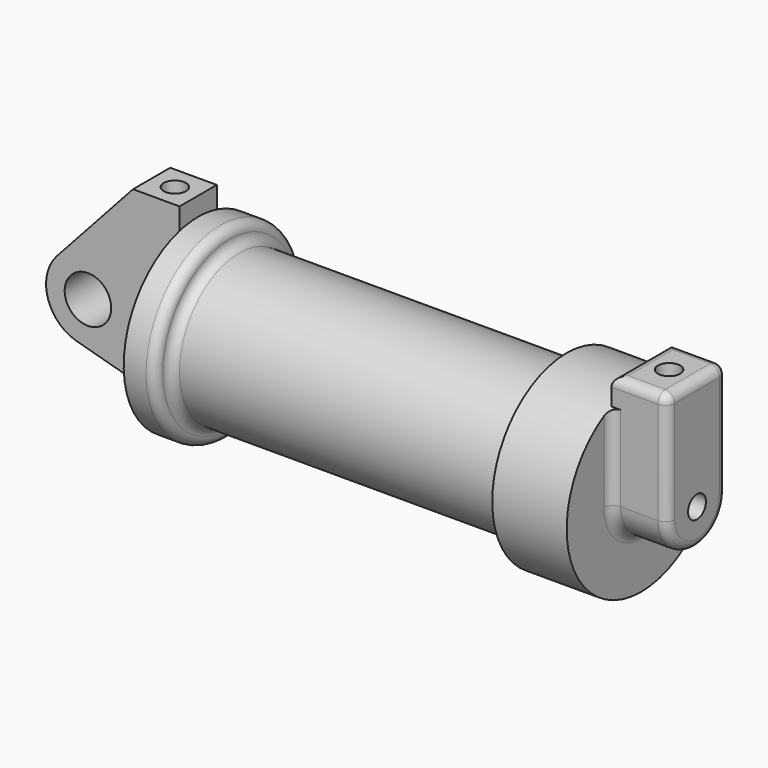
from build123d import *

# Parameters (mm, degrees)
F0_W          = 5.842
F0_H          = 12.7
F0_R          = 3.175
F2_DEPTH      = 3.175
F3_R          = 1.524
F4_DEPTH      = 7.62
F5_R          = 1.524
F7_DEPTH      = 17.78
F6_R          = 1.524
F8_DEPTH      = 10.414
F9_R          = 1.26999
F10_T4_DEPTH  = 14.8147422652
F10_S5_R      = 12.7
F10_T6_DEPTH  = 9
F10_T10_DEPTH = 14.8147422652
F10_S11_R     = 12.7
F10_T12_DEPTH = 9
F10_T14_ANGLE = 180
F10_T15_DEPTH = 13.97
F10_T17_DEPTH = 7.62
F10_T19_DEPTH = 16.51
F10_T21_DEPTH = 9.525
F10_S25_W     = 1.2954
F10_S25_H     = 1.2954
F10_T26_DEPTH = 1.2954
F10_S31_W     = 1.2954
F10_S31_H     = 1.2954
F10_T32_DEPTH = 1.2954
F10_T36_ANGLE = 180


# Not quite as in the source:
# - a fillet or chamfer that OpenCascade refuses, or shapes differently, is made with other operations: its cross-section is extruded or revolved along the edge and cut away or added
# - a fillet or chamfer is up to 0.001 mm smaller than in the source, because OpenCascade refuses the exact size


with BuildPart() as f1:
    # F0 (on Front) → F1 (revolve)
    with BuildSketch(Plane.XZ):
        Polygon((5.842, 12.7), (5.842, 0), (66.294, 0), (66.294, 12.7), (56.134, 12.7), (56.134, 10.16), (10.16, 10.16), (10.16, 12.7), align=None)
    revolve(axis=Axis((33.147, 0, 0), (-1, 0, 0)))

    # F0 (on Front) → F2 (join, symmetric)
    with BuildSketch(Plane.XZ):
        with BuildLine():
            Line((5.842, 0), (0, 0))
            Line((0, 0), (-0.9398, 0))
            ThreePointArc((-0.9398, 0), (-3.1957909266, -4.5493385486), (-8.1826630726, -5.5069827884))
            Line((-8.1826630726, -5.5069827884), (5.842, -9.398))
            Line((5.842, -9.398), (5.842, 0))
        make_face()
        with BuildLine():
            Line((-0.9398, 0), (0, 0))
            Line((0, 0), (0, 12.7))
            Line((0, 12.7), (5.842, 12.7))
            Line((5.842, 12.7), (5.842, 15.24))
            Line((5.842, 15.24), (-0.508, 15.24))
            Line((-0.508, 15.24), (-10.8806298187, 3.8475430269))
            ThreePointArc((-10.8806298187, 3.8475430269), (-4.5919612295, 5.3297205562), (-0.9398, 0))
        make_face()
        with Locations((2.921, 6.35)):
            Rectangle(F0_W, F0_H)
        with BuildLine():
            ThreePointArc((-8.1826630726, -5.5069827884), (-3.1957909266, -4.5493385486), (-0.9398, 0))
            ThreePointArc((-0.9398, 0), (-4.5919612295, 5.3297205562), (-10.8806298187, 3.8475430269))
            ThreePointArc((-10.8806298187, 3.8475430269), (-12.1459778134, -1.5837270034), (-8.1826630726, -5.5069827884))
        make_face()
        with Locations((-6.6548, 0)):
            Circle(F0_R, mode=Mode.SUBTRACT)
    extrude(amount=F2_DEPTH, both=True)

    # F3 (on face) → F4 (join)
    with BuildSketch(Plane.YZ.offset(66.294)):
        with BuildLine():
            ThreePointArc((-5.08, 0), (0, -5.08), (5.08, 0))
            ThreePointArc((5.08, 0), (0, 5.08), (-5.08, 0))
        make_face()
        Circle(F3_R, mode=Mode.SUBTRACT)
        with BuildLine():
            ThreePointArc((-5.08, 0), (0, 5.08), (5.08, 0))
            Line((5.08, 0), (5.08, 15.24))
            Line((5.08, 15.24), (-5.08, 15.24))
            Line((-5.08, 15.24), (-5.08, 0))
        make_face()
    extrude(amount=F4_DEPTH)

    # F5 (on face) → F7 (cut)
    with BuildSketch(Plane.XY.offset(15.24)):
        with Locations((2.667, 0)):
            Circle(F5_R)
    extrude(amount=-F7_DEPTH, mode=Mode.SUBTRACT)

    # F6 (on face) → F8 (cut)
    with BuildSketch(Plane.XY.offset(15.24)):
        with Locations((70.104, 0)):
            Circle(F6_R)
    extrude(amount=-F8_DEPTH, mode=Mode.SUBTRACT)

    # F9 (radius 1.27 in the source; OpenCascade refuses exactly that, so slightly less here)
    f9_edges = [f1.edges().sort_by_distance(p)[0] for p in [
        (10.16, 0, -12.7),
        (10.16, 0, -10.16),
    ]]
    fillet(f9_edges, radius=F9_R)

    # F10: fillet of radius 1.27 on 12 edges, made by hand


with BuildPart() as f10_tool2:
    # F10_s3 → F10_t4 (new body)
    with BuildSketch(Plane.XY.offset(14.8147422652)):
        with BuildLine():
            ThreePointArc((66.294, -6.35), (66.6659743879, -5.4519743879), (67.564, -5.08))
            Line((67.564, -5.08), (66.294, -5.08))
            Line((66.294, -5.08), (66.294, -6.35))
        make_face()
    extrude(amount=-F10_T4_DEPTH)

    # F10_s5 → F10_t6 (intersect, symmetric)
    with BuildSketch(Plane.YZ.offset(66.9)):
        Circle(F10_S5_R)
    extrude(amount=F10_T6_DEPTH, both=True, mode=Mode.INTERSECT)


with BuildPart() as f1_1:
    add(f1.part)

    # F10_t1: union F10_tool2
    add(f10_tool2.part)


with BuildPart() as f10_tool8:
    # F10_s9 → F10_t10 (new body)
    with BuildSketch(Plane.XY):
        with BuildLine():
            ThreePointArc((66.294, 6.35), (66.6659743879, 5.4519743879), (67.564, 5.08))
            Line((67.564, 5.08), (66.294, 5.08))
            Line((66.294, 5.08), (66.294, 6.35))
        make_face()
    extrude(amount=F10_T10_DEPTH)

    # F10_s11 → F10_t12 (intersect, symmetric)
    with BuildSketch(Plane.YZ.offset(66.9)):
        Circle(F10_S11_R)
    extrude(amount=F10_T12_DEPTH, both=True, mode=Mode.INTERSECT)


with BuildPart() as f1_2:
    add(f1_1.part)

    # F10_t7: union F10_tool8
    add(f10_tool8.part)

    # F10_s13 → F10_t14 (revolve)
    with BuildSketch(Plane.XY):
        with BuildLine():
            ThreePointArc((66.294, -6.35), (66.6659743879, -5.4519743879), (67.564, -5.08))
            Line((67.564, -5.08), (66.294, -5.08))
            Line((66.294, -5.08), (66.294, -6.35))
        make_face()
    revolve(axis=Axis((66.294, 0, 0), (1, 0, 0)), revolution_arc=F10_T14_ANGLE)

    # F10_s16 → F10_t15 (cut)
    with BuildSketch(Plane.XY):
        with BuildLine():
            ThreePointArc((72.644, 5.08), (73.5420256121, 4.7080256121), (73.914, 3.81))
            Line((73.914, 3.81), (73.914, 5.08))
            Line((73.914, 5.08), (72.644, 5.08))
        make_face()
        with BuildLine():
            ThreePointArc((72.644, -5.08), (73.5420256121, -4.7080256121), (73.914, -3.81))
            Line((73.914, -3.81), (73.914, -5.08))
            Line((73.914, -5.08), (72.644, -5.08))
        make_face()
    extrude(amount=F10_T15_DEPTH, mode=Mode.SUBTRACT)

    # F10_s18 → F10_t17 (cut)
    with BuildSketch(Plane.XZ.offset(-3.81)):
        with BuildLine():
            ThreePointArc((72.644, 15.24), (73.5420256121, 14.8680256121), (73.914, 13.97))
            Line((73.914, 13.97), (73.914, 15.24))
            Line((73.914, 15.24), (72.644, 15.24))
        make_face()
    extrude(amount=F10_T17_DEPTH, mode=Mode.SUBTRACT)

    # F10_s20 → F10_t19 (cut)
    with BuildSketch(Plane.XZ.offset(-8.255)):
        with BuildLine():
            ThreePointArc((66.294, 13.97), (66.6659743879, 14.8680256121), (67.564, 15.24))
            Line((67.564, 15.24), (66.294, 15.24))
            Line((66.294, 15.24), (66.294, 13.97))
        make_face()
    extrude(amount=F10_T19_DEPTH, mode=Mode.SUBTRACT)

    # F10_s22 → F10_t21 (cut)
    with BuildSketch(Plane.YZ.offset(63.119)):
        with BuildLine():
            ThreePointArc((3.81, 15.24), (4.7080256121, 14.8680256121), (5.08, 13.97))
            Line((5.08, 13.97), (5.08, 15.24))
            Line((5.08, 15.24), (3.81, 15.24))
        make_face()
        with BuildLine():
            ThreePointArc((-5.08, 13.97), (-4.7080256121, 14.8680256121), (-3.81, 15.24))
            Line((-3.81, 15.24), (-5.08, 15.24))
            Line((-5.08, 15.24), (-5.08, 13.97))
        make_face()
    extrude(amount=F10_T21_DEPTH, mode=Mode.SUBTRACT)


with BuildPart() as f10_tool24:
    # F10_s25 → F10_t26 (new body)
    with BuildSketch(Plane.XY.offset(13.97)):
        with Locations((73.2917, 4.4577)):
            Rectangle(F10_S25_W, F10_S25_H)
    extrude(amount=F10_T26_DEPTH)

    # F10_s27 → F10_t28 (revolve, cut)
    with BuildSketch(Plane(origin=(72.644, 3.81, 13.97), x_dir=(-0.7071067812, -0.7071067812, 0), z_dir=(-0.7071067812, 0.7071067812, 0))):
        with BuildLine():
            ThreePointArc((0, -1.27), (1.27, 0), (0, 1.27))
            Line((0, 1.27), (0, -1.27))
        make_face()
    revolve(axis=Axis((72.644, 3.81, 13.97), (0, 0, 1)), mode=Mode.SUBTRACT)


with BuildPart() as f1_3:
    add(f1_2.part)

    # F10_t23: cut F10_tool24
    add(f10_tool24.part, mode=Mode.SUBTRACT)


with BuildPart() as f10_tool30:
    # F10_s31 → F10_t32 (new body)
    with BuildSketch(Plane.XZ.offset(3.81)):
        with Locations((73.2917, 14.6177)):
            Rectangle(F10_S31_W, F10_S31_H)
    extrude(amount=F10_T32_DEPTH)

    # F10_s33 → F10_t34 (revolve, cut)
    with BuildSketch(Plane(origin=(72.644, -3.81, 13.97), x_dir=(-0.7071067812, 0, -0.7071067812), z_dir=(-0.7071067812, 0, 0.7071067812))):
        with BuildLine():
            ThreePointArc((0, -1.27), (1.27, 0), (0, 1.27))
            Line((0, 1.27), (0, -1.27))
        make_face()
    revolve(axis=Axis((72.644, -3.81, 13.97), (0, -1, 0)), mode=Mode.SUBTRACT)


with BuildPart() as f1_4:
    add(f1_3.part)

    # F10_t29: cut F10_tool30
    add(f10_tool30.part, mode=Mode.SUBTRACT)

    # F10_s35 → F10_t36 (revolve, cut)
    with BuildSketch(Plane.XY):
        with BuildLine():
            ThreePointArc((72.644, -5.08), (73.5420256121, -4.7080256121), (73.914, -3.81))
            Line((73.914, -3.81), (73.914, -5.08))
            Line((73.914, -5.08), (72.644, -5.08))
        make_face()
    revolve(axis=Axis((73.914, 0, 0), (1, 0, 0)), revolution_arc=F10_T36_ANGLE, mode=Mode.SUBTRACT)


solid = f1_4.part
